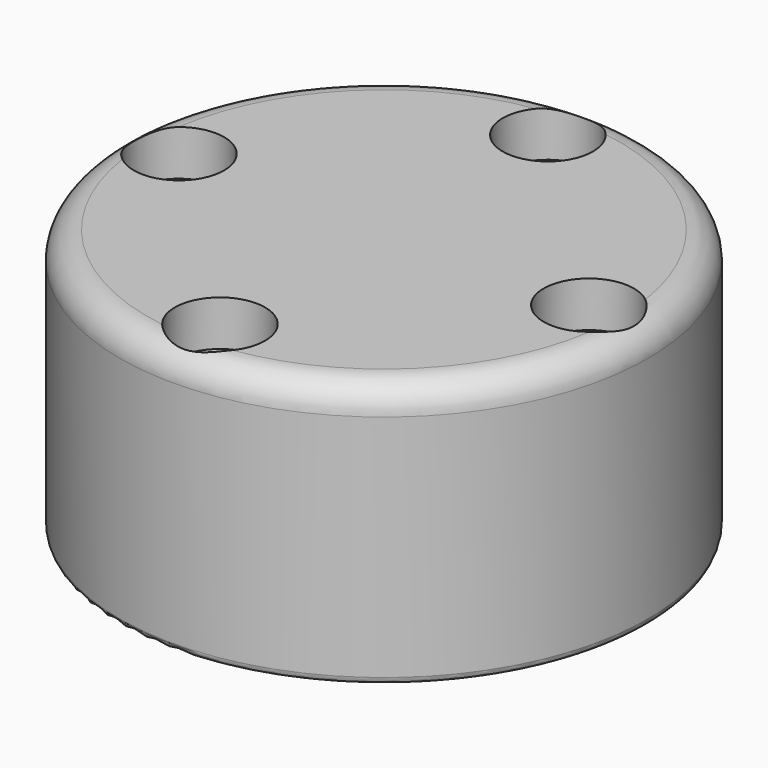
from build123d import *

# Parameters (mm, degrees)
F3_D           = 3.3
F3_DEPTH       = 8
F3_START       = 0.2679493
F3_CBORE_D     = 6.5
F3_CBORE_DEPTH = 3
F3_TIP         = 0.9914200214


with BuildPart() as f1:
    # F0 (on Front) → F1 (revolve)
    with BuildSketch(Plane.XZ):
        with BuildLine():
            Line((-16.5, 0), (0, 0))
            Line((0, 0), (0, 5))
            Line((0, 5), (-17, 5))
            ThreePointArc((-17, 5), (-18.4142135624, 4.4142135624), (-19, 3))
            Line((-19, 3), (-19, -13.5))
            ThreePointArc((-19, -13.5), (-18.8535533906, -13.8535533906), (-18.5, -14))
            Line((-18.5, -14), (-17, -14))
            Line((-17, -14), (-17, -0.5))
            ThreePointArc((-17, -0.5), (-16.8535533906, -0.1464466094), (-16.5, 0))
        make_face()
    revolve(axis=Axis((0, 0, 2.5), (0, 0, 1)))

    # F3
    # its depths count from where the whole tool has entered the part; down to there all is cleared
    with Locations(Plane.XY.offset(5).offset(-F3_START)):
        with Locations((0, 14.75), (14.75, 0), (0, -14.75), (-14.75, 0)):
            CounterBoreHole(F3_D / 2, F3_CBORE_D / 2, F3_CBORE_DEPTH, depth=F3_DEPTH)
            with Locations((0, 0, -(F3_DEPTH + F3_TIP / 2))):  # 118° drill point
                Cone(0, F3_D / 2, F3_TIP, mode=Mode.SUBTRACT)


solid = f1.part
